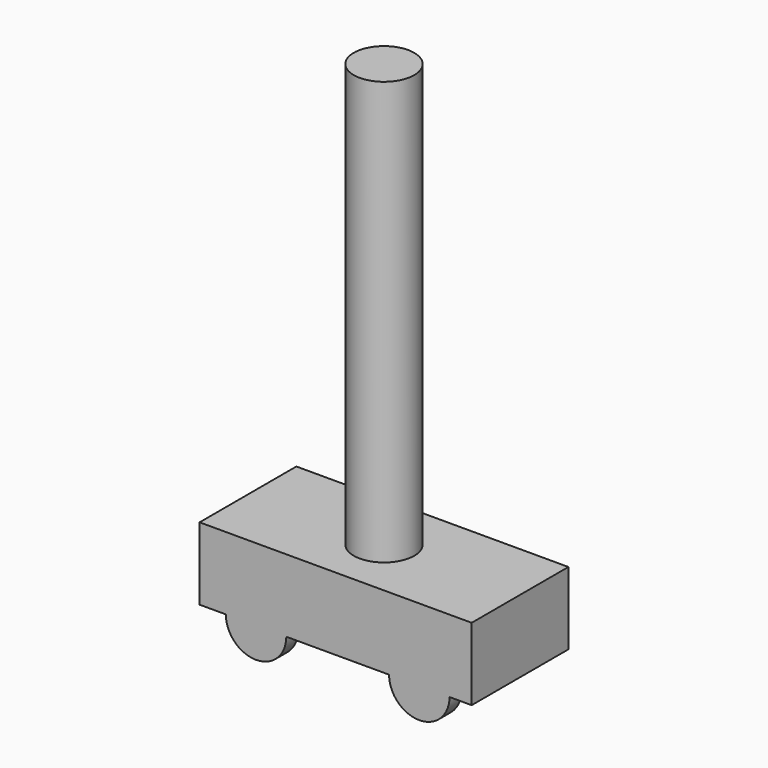
from build123d import *

# Parameters (mm, degrees)
F0_W     = 114.3
F0_H     = 50.8
F1_DEPTH = 30.48
F2_R     = 12.7
F3_DEPTH = 177.8
F5_DEPTH = 6.35
F7_DEPTH = 6.35


with BuildPart() as f1:
    # F0 (on Top) → F1 (new body)
    with BuildSketch(Plane.XY):
        Rectangle(F0_W, F0_H)
    extrude(amount=F1_DEPTH)

    # F2 (on face) → F3 (join)
    with BuildSketch(Plane.XY.offset(30.48)):
        Circle(F2_R)
    extrude(amount=F3_DEPTH)

    # F4 (on face) → F5 (join)
    with BuildSketch(Plane(origin=(0, 25.4, 0), x_dir=(-1, 0, 0), z_dir=(0, 1, 0))):
        with BuildLine():
            Line((-47.841646862, 0), (-22.441646862, 0))
            ThreePointArc((-22.441646862, 0), (-35.141646862, 12.7), (-47.841646862, 0))
        make_face()
        with BuildLine():
            ThreePointArc((-47.841646862, 0), (-35.141646862, -12.7), (-22.441646862, 0))
            Line((-22.441646862, 0), (-47.841646862, 0))
        make_face()
        with BuildLine():
            Line((46.138353138, 0), (20.738353138, 0))
            ThreePointArc((20.738353138, 0), (33.438353138, -12.7), (46.138353138, 0))
        make_face()
    extrude(amount=-F5_DEPTH)

    # F6 (on face) → F7 (join)
    with BuildSketch(Plane.XZ.offset(25.4)):
        with BuildLine():
            ThreePointArc((-46.1274172783, 0), (-33.4274172783, -12.7), (-20.7274172783, 0))
            Line((-20.7274172783, 0), (-46.1274172783, 0))
        make_face()
        with BuildLine():
            Line((47.8525827217, 0), (22.4525827217, 0))
            ThreePointArc((22.4525827217, 0), (35.1525827217, -12.7), (47.8525827217, 0))
        make_face()
        with BuildLine():
            ThreePointArc((47.8525827217, 0), (35.1525827217, 12.7), (22.4525827217, 0))
            Line((22.4525827217, 0), (47.8525827217, 0))
        make_face()
    extrude(amount=-F7_DEPTH)


solid = f1.part
